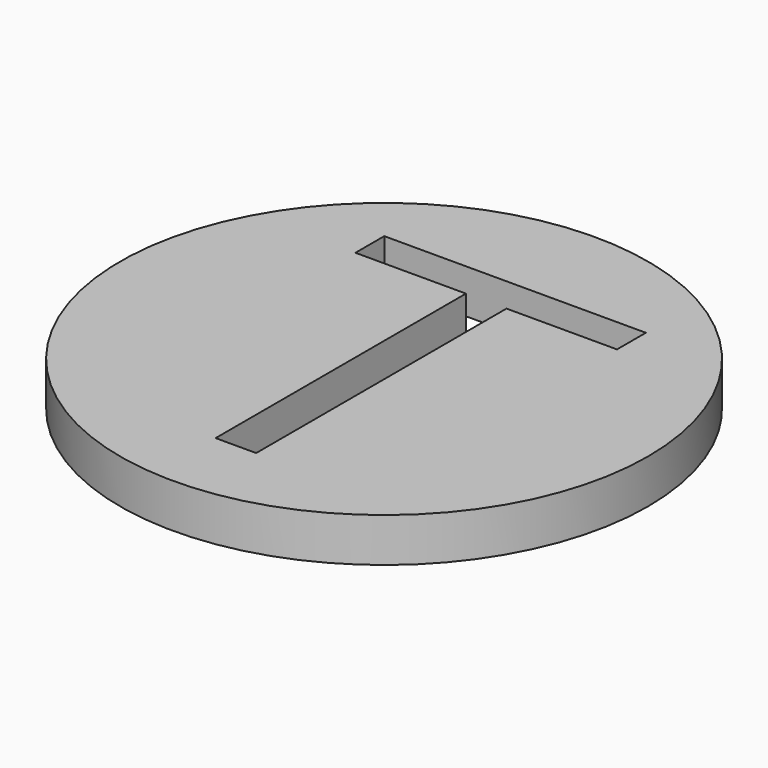
from build123d import *

# Parameters (mm, degrees)
F0_R         = 12
F1_DEPTH     = 2
F2_TEXT_SIZE = 22.2222222222
F3_DEPTH     = 25


# Not quite as in the source:
# - Text() gives the source's letters only with a copy of the font that has no kerning and outlines rounded to 1/6400 em; it was checked with that copy


with BuildPart() as f1:
    # F0 (on Top) → F1 (new body)
    with BuildSketch(Plane.XY):
        Circle(F0_R)
    extrude(amount=F1_DEPTH)

    # F2 (on face) → F3 (cut)
    with BuildSketch(Plane.XY.offset(2)):
        with Locations((-6.089605391, -8.485307917)):
            Text('T', F2_TEXT_SIZE, font='Open Sans', text_align=(TextAlign.LEFT, TextAlign.BOTTOM))
    extrude(amount=-F3_DEPTH, mode=Mode.SUBTRACT)


solid = f1.part
